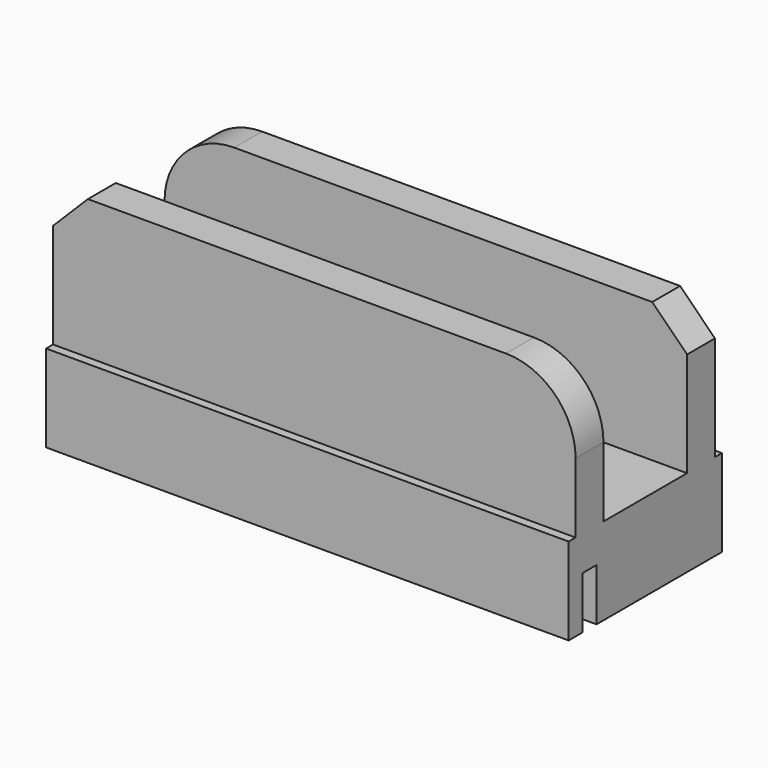
from build123d import *

# Parameters (mm, degrees)
F0_W      = 150
F0_H      = 65
F1_DEPTH  = 55
F2_W      = 5
F2_H      = 15
F3_DEPTH  = 150.001
F4_W      = 30
F4_H      = 40
F5_DEPTH  = 150.001
F6_SIZE   = 10
F7_R      = 20
F8_W      = 2.5
F8_H      = 43.3062759042
F9_DEPTH  = 150.001
F10_W     = 2.5
F10_H     = 43.4678007662
F11_DEPTH = 150.001
F12_R     = 15
F13_DEPTH = 25.001


with BuildPart() as f1:
    # F0 (on Front) → F1 (new body)
    with BuildSketch(Plane.XZ):
        Rectangle(F0_W, F0_H)
    extrude(amount=F1_DEPTH)

    # F2 (on face) → F3 (cut, through all)
    with BuildSketch(Plane.YZ.offset(75)):
        with Locations((-47.5, -25)):
            Rectangle(F2_W, F2_H)
    extrude(amount=-F3_DEPTH, mode=Mode.SUBTRACT)

    # F4 (on face) → F5 (cut, through all)
    with BuildSketch(Plane.YZ.offset(75)):
        with Locations((-27.5, 12.5)):
            Rectangle(F4_W, F4_H)
    extrude(amount=-F5_DEPTH, mode=Mode.SUBTRACT)

    # F6
    f6_edges = [f1.edges().sort_by_distance(p)[0] for p in [
        (75, -6.25, 32.5),
        (-75, -48.75, 32.5),
    ]]
    chamfer(f6_edges, length=F6_SIZE)

    # F7
    f7_edges = [f1.edges().sort_by_distance(p)[0] for p in [
        (75, -48.75, 32.5),
        (-75, -6.25, 32.5),
    ]]
    fillet(f7_edges, radius=F7_R)

    # F8 (on face) → F9 (cut, through all)
    with BuildSketch(Plane.YZ.offset(75)):
        with Locations((-53.75, 14.1531379521)):
            Rectangle(F8_W, F8_H)
    extrude(amount=-F9_DEPTH, mode=Mode.SUBTRACT)

    # F10 (on face) → F11 (cut, through all)
    with BuildSketch(Plane.YZ.offset(75)):
        with Locations((-1.25, 14.2339003831)):
            Rectangle(F10_W, F10_H)
    extrude(amount=-F11_DEPTH, mode=Mode.SUBTRACT)

    # F12 (on face) → F13 (cut, through all)
    with BuildSketch(Plane.XY.offset(-7.5)):
        with Locations((0, -27.5)):
            Circle(F12_R)
    extrude(amount=-F13_DEPTH, mode=Mode.SUBTRACT)


solid = f1.part
